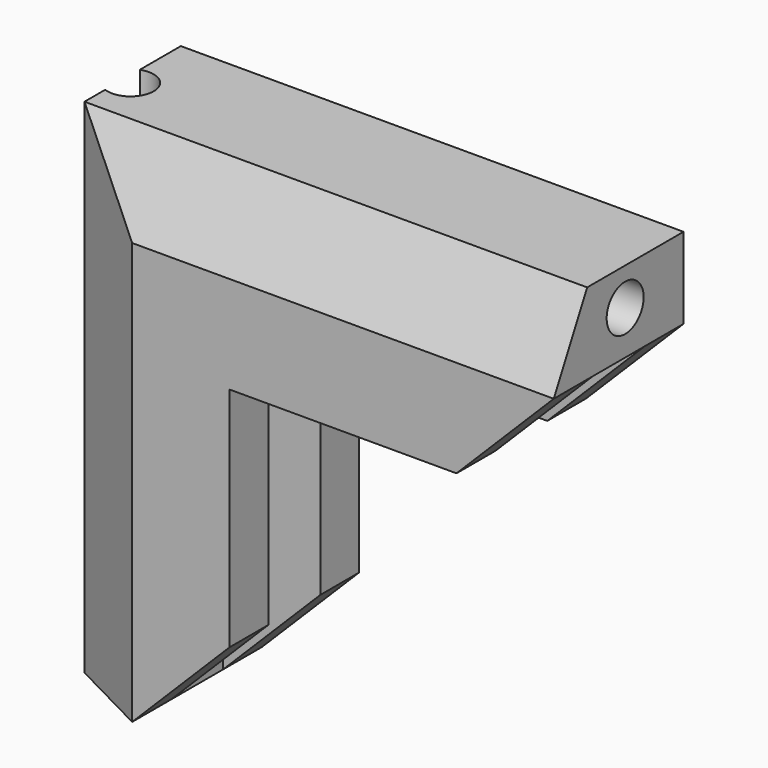
from build123d import *

# Parameters (mm, degrees)
F1_DEPTH      = 20
F2_W          = 7
F2_H          = 20
F3_DEPTH      = 2
F5_DEPTH      = 6
F6_W          = 3
F6_H          = 6
F7_DEPTH      = 25
F8_DEPTH      = 3
F12_DEPTH     = 2
F13_DEPTH     = 11
F14_T4_DEPTH  = 29
F14_T10_DEPTH = 28
F14_T17_DEPTH = 38.2867319519
F14_T24_DEPTH = 39.2867319519
F15_T1_DEPTH  = 61.1449358039
F15_T3_DEPTH  = 60.1449358039
F16_DEPTH     = 1
F17_SIZE      = 6
F20_D         = 2.85
F20_ON_F18_D  = 2.85
F22_DEPTH     = 3
F24_D         = 6.5
F24_DEPTH     = 2
F24_TIP       = 1.9527970118


# Not quite as in the source:
# - a fillet or chamfer that OpenCascade refuses, or shapes differently, is made with other operations: its cross-section is extruded or revolved along the edge and cut away or added


with BuildPart() as f1:
    # F0 (on Top) → F1 (new body)
    with BuildSketch(Plane.XY):
        Polygon((-3.1551690071, 9.1141472052), (-12.1551690071, 9.1141472052), (-12.1551690071, -0.8858527948), (-3.1551690071, -0.8858527948), (-3.1551690071, 2.1141472052), (-9.1551690071, 2.1141472052), (-9.1551690071, 6.1141472052), (-3.1551690071, 6.1141472052), align=None)
    extrude(amount=F1_DEPTH)

    # F2 (on face) → F3 (join)
    with BuildSketch(Plane(origin=(-12.1551690071, 0, 0), x_dir=(0, -1, 0), z_dir=(-1, 0, 0))):
        with Locations((-5.6141472052, 10)):
            Rectangle(F2_W, F2_H)
    extrude(amount=F3_DEPTH)

    # F4 (on face) → F5 (join)
    with BuildSketch(Plane.XY.offset(20)):
        Polygon((-12.1345976368, 9.1141472052), (-12.1551690071, 2.1141472052), (-12.1551690071, -0.8858527948), (-9.1551690071, -0.8858527948), (-9.1551690071, 2.1141472052), (-9.1551690071, 6.1141472052), (-9.1551690071, 9.1141472052), align=None)
    extrude(amount=F5_DEPTH)

    # F6 (on face) → F7 (join)
    with BuildSketch(Plane.YZ.offset(-9.1551690071)):
        with Locations((7.6141472052, 23)):
            Rectangle(F6_W, F6_H)
        with Locations((0.6141472052, 23)):
            Rectangle(F6_W, F6_H)
        Polygon((-0.8858527948, 26), (2.1141472052, 26), (6.1141472052, 26), (9.1141472052, 26), (9.1141472052, 29), (-0.8858527948, 29), align=None)
    extrude(amount=F7_DEPTH)

    # F8 (add): a face of the model
    f8_faces = [f1.faces().sort_by_distance(p)[0] for p in [
        (-10.6515768532, 4.1077318265, 26),
    ]]
    extrude(f8_faces, amount=F8_DEPTH)

    # F9: union 

    # F10: union 

    # F11 (on face) → F12 (join)
    with BuildSketch(Plane.XY.offset(29)):
        Polygon((-12.1345976368, 9.1141472052), (-12.1551690071, 2.1141472052), (15.8448309929, 2.1141472052), (15.8448309929, 9.1141472052), align=None)
    extrude(amount=F12_DEPTH)

    # F4 (on face) → F13 (join)
    with BuildSketch(Plane.XY.offset(20)):
        Polygon((-14.1551690071, 2.1141472052), (-12.1551690071, 2.1141472052), (-12.1345976368, 9.1141472052), (-14.1551690071, 9.1141472052), align=None)
    extrude(amount=F13_DEPTH)

    # F14: chamfer of 4 on 2 edges, made by hand


with BuildPart() as f14_tool2:
    # F14_s3 → F14_t4 (new body)
    with BuildSketch(Plane.XY):
        Polygon((-12.1551690071, -1.8858527948), (-16.1551690071, 2.1141472052), (-12.1551690071, 2.1141472052), align=None)
    extrude(amount=F14_T4_DEPTH)

    split(bisect_by=Plane.XZ.offset(0.8858527948), keep=Keep.BOTTOM)

    split(bisect_by=Plane.YZ.offset(-14.1551690071), keep=Keep.TOP)


with BuildPart() as f1_1:
    add(f1.part)

    # F14_t1: union F14_tool2
    add(f14_tool2.part)


with BuildPart() as f14_tool8:
    # F14_s9 → F14_t10 (new body)
    with BuildSketch(Plane.YZ.offset(-12.1551690071)):
        Polygon((-1.8858527948, 29), (2.1141472052, 33), (2.1141472052, 29), align=None)
    extrude(amount=F14_T10_DEPTH)

    split(bisect_by=Plane.XZ.offset(0.8858527948), keep=Keep.BOTTOM)

    split(bisect_by=Plane.XY.offset(31), keep=Keep.BOTTOM)


with BuildPart() as f1_2:
    add(f1_1.part)

    # F14_t7: union F14_tool8
    add(f14_tool8.part)


with BuildPart() as f14_tool15:
    # F14_s16 → F14_t17 (new body)
    with BuildSketch(Plane.YZ.offset(-22.4419009589)):
        Polygon((-1.8858527948, 29), (2.1141472052, 33), (2.1141472052, 29), align=None)
    extrude(amount=F14_T17_DEPTH)

    split(bisect_by=Plane.XZ.offset(0.8858527948), keep=Keep.BOTTOM)

    split(bisect_by=Plane.YZ.offset(-12.1551690071), keep=Keep.BOTTOM)

    split(bisect_by=Plane.YZ.offset(-14.1551690071), keep=Keep.TOP)

    split(bisect_by=Plane.XY.offset(31), keep=Keep.BOTTOM)


with BuildPart() as f14_tool22:
    # F14_s23 → F14_t24 (new body)
    with BuildSketch(Plane.XY):
        Polygon((-12.1551690071, -1.8858527948), (-16.1551690071, 2.1141472052), (-12.1551690071, 2.1141472052), align=None)
    extrude(amount=F14_T24_DEPTH)

    split(bisect_by=Plane.XZ.offset(0.8858527948), keep=Keep.BOTTOM)

    split(bisect_by=Plane.XY.offset(29), keep=Keep.TOP)

    split(bisect_by=Plane.YZ.offset(-14.1551690071), keep=Keep.TOP)

    split(bisect_by=Plane.XY.offset(31), keep=Keep.BOTTOM)


with BuildPart() as f14_tool15_1:
    add(f14_tool15.part)

    # F14_t29: intersect F14_tool22
    add(f14_tool22.part, mode=Mode.INTERSECT)


with BuildPart() as f1_3:
    add(f1_2.part)

    # F14_t13: union F14_tool15
    add(f14_tool15_1.part)

    # F15: chamfer of 4 x 6 on 2 edges, made by hand

    # F15_s2 → F15_t1 (cut)
    with BuildSketch(Plane.XY.offset(-15.5724679019)):
        Polygon((-9.1551690071, -0.8858527948), (-17.3978096942, 3.3567878923), (-13.1551690071, -0.8858527948), align=None)
    extrude(amount=F15_T1_DEPTH, mode=Mode.SUBTRACT)

    # F15_s4 → F15_t3 (cut)
    with BuildSketch(Plane.YZ.offset(-28.7276369091)):
        Polygon((-0.8858527948, 26), (3.3567878923, 34.2426406871), (-0.8858527948, 30), align=None)
    extrude(amount=F15_T3_DEPTH, mode=Mode.SUBTRACT)

    # F16 (add): a face of the model
    f16_faces = [f1_3.faces().sort_by_distance(p)[0] for p in [
        (15.8448309929, 6.2628078927, 23),
    ]]
    extrude(f16_faces, amount=F16_DEPTH)

    # F17
    f17_edges = [f1_3.edges().sort_by_distance(p)[0] for p in [
        (-3.155169, 0.614147, 0),
        (-3.155169, 7.614147, 0),
        (16.844831, 0.614147, 20),
        (16.844831, 7.614147, 20),
    ]]
    chamfer(f17_edges, length=F17_SIZE)

    # F20 (through all)
    with Locations(Plane(origin=(0, 0, 0), x_dir=(1, 0, 0), z_dir=(0, 0, -1))):
        with Locations((-13.6551690071, -4.6141472052)):
            Hole(F20_D / 2)

    # F20 on F18 (through all)
    with Locations(Plane.YZ.offset(16.8448309929)):
        with Locations((4.6141472052, 28.7)):
            Hole(F20_ON_F18_D / 2)

    # F21 (on face) → F22 (cut)
    with BuildSketch(Plane(origin=(0, 9.1141472052, 0), x_dir=(-1, 0, 0), z_dir=(0, 1, 0))):
        with BuildLine():
            ThreePointArc((10.2461592647, 27.0909902577), (7.0641787494, 27.0909902577), (7.0641787494, 23.9090097423))
            Line((7.0641787494, 23.9090097423), (10.2461592647, 27.0909902577))
        make_face()
        with BuildLine():
            Line((10.2461592647, 27.0909902577), (7.0641787494, 23.9090097423))
            ThreePointArc((7.0641787494, 23.9090097423), (9.5162067299, 23.4212710518), (10.9051690071, 25.5))
            ThreePointArc((10.9051690071, 25.5), (10.7338979552, 26.3610377228), (10.2461592647, 27.0909902577))
        make_face()
    extrude(amount=-F22_DEPTH, mode=Mode.SUBTRACT)

    # F24 (one way)
    with BuildSketch(Plane(origin=(0, 6.1141472052, 0), x_dir=(-1, 0, 0), z_dir=(0, -1, 0))):
        with Locations((8.6551690071, -25.5)):
            Circle(F24_D / 2)
    extrude(amount=-F24_DEPTH, mode=Mode.SUBTRACT)
    with Locations(Plane(origin=(0, 6.1141472052, 0), x_dir=(-1, 0, 0), z_dir=(0, -1, 0))):
        with Locations((8.6551690071, -25.5)):
            with Locations((0, 0, -(F24_DEPTH + F24_TIP / 2))):  # 118° drill point
                Cone(0, F24_D / 2, F24_TIP, mode=Mode.SUBTRACT)


solid = f1_3.part
